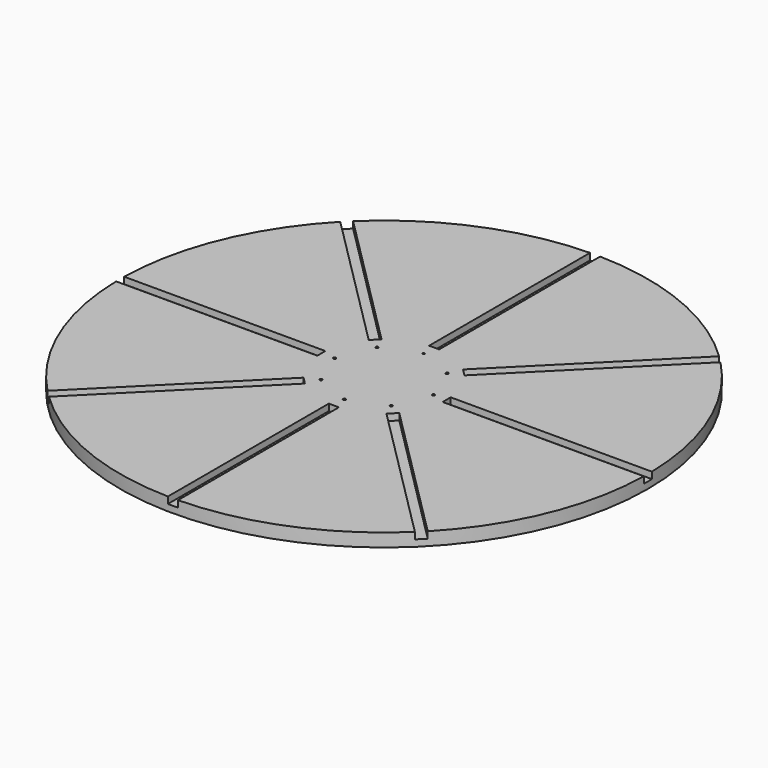
from build123d import *

# Parameters (mm, degrees)
F0_R      = 400
F1_DEPTH  = 20
F3_R      = 2
F4_DEPTH  = 20
F5_R      = 2
F6_DEPTH  = 20
F8_R      = 2
F9_DEPTH  = 20
F10_R     = 2
F11_DEPTH = 20
F12_R     = 2
F13_DEPTH = 20
F14_R     = 2
F15_DEPTH = 20
F16_R     = 1.4677946232
F17_DEPTH = 20
F18_R     = 2
F19_DEPTH = 20
F20_W     = 15.2905675913
F20_H     = 305
F20_W_2   = 305
F20_H_2   = 15.2905675913
F21_DEPTH = 10


with BuildPart() as f1:
    # F0 (on Top) → F1 (new body)
    with BuildSketch(Plane.XY):
        Circle(F0_R)
    extrude(amount=-F1_DEPTH)

    # F3 (on Top) → F4 (cut)
    with BuildSketch(Plane.XY):
        with Locations((-75, 0)):
            Circle(F3_R)
    extrude(amount=-F4_DEPTH, mode=Mode.SUBTRACT)

    # F5 (on Top) → F6 (cut)
    with BuildSketch(Plane.XY):
        with Locations((-53.1572374294, -52.9084880607)):
            Circle(F5_R)
    extrude(amount=-F6_DEPTH, mode=Mode.SUBTRACT)

    # F8 (on offset) → F9 (cut)
    with BuildSketch(Plane.XY):
        with Locations((0, -75)):
            Circle(F8_R)
    extrude(amount=-F9_DEPTH, mode=Mode.SUBTRACT)

    # F10 (on offset) → F11 (cut)
    with BuildSketch(Plane.XY):
        with Locations((53.3727891743, -52.9747456312)):
            Circle(F10_R)
    extrude(amount=-F11_DEPTH, mode=Mode.SUBTRACT)

    # F12 (on offset) → F13 (cut)
    with BuildSketch(Plane.XY):
        with Locations((75, 0)):
            Circle(F12_R)
    extrude(amount=-F13_DEPTH, mode=Mode.SUBTRACT)

    # F14 (on offset) → F15 (cut)
    with BuildSketch(Plane.XY):
        with Locations((53.0946776271, 53.1038790941)):
            Circle(F14_R)
    extrude(amount=-F15_DEPTH, mode=Mode.SUBTRACT)

    # F16 (on offset) → F17 (cut)
    with BuildSketch(Plane.XY):
        with Locations((0, 75)):
            Circle(F16_R)
    extrude(amount=-F17_DEPTH, mode=Mode.SUBTRACT)

    # F18 (on offset) → F19 (cut)
    with BuildSketch(Plane.XY):
        with Locations((-53.0560910702, 53.0486702919)):
            Circle(F18_R)
    extrude(amount=-F19_DEPTH, mode=Mode.SUBTRACT)

    # F20 (on offset) → F21 (cut)
    with BuildSketch(Plane.XY):
        with Locations((0, -247.5)):
            Rectangle(F20_W, F20_H)
        Polygon((288.2487444906, -277.4366804586), (72.5811762287, -61.7691121967), (61.7691121967, -72.5811762287), (277.4366804586, -288.2487444906), align=None)
        with Locations((247.5, 0)):
            Rectangle(F20_W_2, F20_H_2)
        Polygon((277.4366804586, 288.2487444906), (61.7691121967, 72.5811762287), (72.5811762287, 61.7691121967), (288.2487444906, 277.4366804586), align=None)
        with Locations((0, 247.5)):
            Rectangle(F20_W, F20_H)
        Polygon((-288.2487444906, 277.4366804586), (-72.5811762287, 61.7691121967), (-61.7691121967, 72.5811762287), (-277.4366804586, 288.2487444906), align=None)
        with Locations((-247.5, 0)):
            Rectangle(F20_W_2, F20_H_2)
        Polygon((-277.4366804586, -288.2487444906), (-61.7691121967, -72.5811762287), (-72.5811762287, -61.7691121967), (-288.2487444906, -277.4366804586), align=None)
    extrude(amount=-F21_DEPTH, mode=Mode.SUBTRACT)


solid = f1.part
